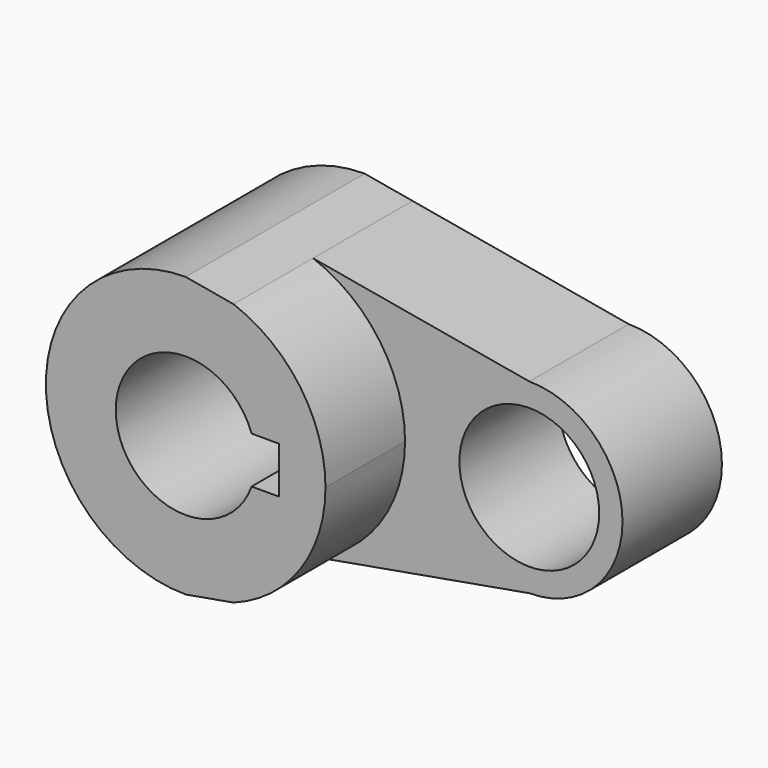
from build123d import *

# Parameters (mm, degrees)
F0_R     = 14.2875
F1_DEPTH = 25.4
F2_DEPTH = 45.72


with BuildPart() as f1:
    # F0 (on Front) → F1 (new body)
    with BuildSketch(Plane.XZ):
        with BuildLine():
            Line((9.780704698, 26.8489932886), (0, 28.575))
            ThreePointArc((0, 28.575), (-28.575, 0), (0, -28.575))
            Line((0, -28.575), (9.780704698, -26.8489932886))
            ThreePointArc((9.780704698, -26.8489932886), (23.4095521288, -16.3866864902), (28.575, 0))
            ThreePointArc((28.575, 0), (23.4095521288, 16.3866864902), (9.780704698, 26.8489932886))
        make_face()
        with BuildLine():
            ThreePointArc((-13.4703841816, 4.7625), (0, 14.2875), (13.4703841816, 4.7625))
            Line((13.4703841816, 4.7625), (19.05, 4.7625))
            Line((19.05, 4.7625), (19.05, -4.7625))
            Line((19.05, -4.7625), (13.4703841816, -4.7625))
            ThreePointArc((13.4703841816, -4.7625), (0, -14.2875), (-13.4703841816, -4.7625))
            Line((-13.4703841816, -4.7625), (-19.05, -4.7625))
            Line((-19.05, -4.7625), (-19.05, 4.7625))
            Line((-19.05, 4.7625), (-13.4703841816, 4.7625))
        make_face(mode=Mode.SUBTRACT)
        with BuildLine():
            Line((53.975, 19.05), (9.780704698, 26.8489932886))
            ThreePointArc((9.780704698, 26.8489932886), (23.4095521288, 16.3866864902), (28.575, 0))
            ThreePointArc((28.575, 0), (23.4095521288, -16.3866864902), (9.780704698, -26.8489932886))
            Line((9.780704698, -26.8489932886), (53.975, -19.05))
            ThreePointArc((53.975, -19.05), (34.925, 0), (53.975, 19.05))
        make_face()
        with BuildLine():
            ThreePointArc((73.025, 0), (67.4453841816, 13.4703841816), (53.975, 19.05))
            ThreePointArc((53.975, 19.05), (34.925, 0), (53.975, -19.05))
            ThreePointArc((53.975, -19.05), (67.4453841816, -13.4703841816), (73.025, 0))
        make_face()
        with Locations((53.975, 0)):
            Circle(F0_R, mode=Mode.SUBTRACT)
        with BuildLine():
            ThreePointArc((-13.4703841816, -4.7625), (-14.2875, 0), (-13.4703841816, 4.7625))
            Line((-13.4703841816, 4.7625), (-19.05, 4.7625))
            Line((-19.05, 4.7625), (-19.05, -4.7625))
            Line((-19.05, -4.7625), (-13.4703841816, -4.7625))
        make_face()
    extrude(amount=F1_DEPTH)

    # F0 (on Front) → F2 (join)
    with BuildSketch(Plane.XZ):
        with BuildLine():
            Line((9.780704698, 26.8489932886), (0, 28.575))
            ThreePointArc((0, 28.575), (-28.575, 0), (0, -28.575))
            Line((0, -28.575), (9.780704698, -26.8489932886))
            ThreePointArc((9.780704698, -26.8489932886), (23.4095521288, -16.3866864902), (28.575, 0))
            ThreePointArc((28.575, 0), (23.4095521288, 16.3866864902), (9.780704698, 26.8489932886))
        make_face()
        with BuildLine():
            ThreePointArc((-13.4703841816, 4.7625), (0, 14.2875), (13.4703841816, 4.7625))
            Line((13.4703841816, 4.7625), (19.05, 4.7625))
            Line((19.05, 4.7625), (19.05, -4.7625))
            Line((19.05, -4.7625), (13.4703841816, -4.7625))
            ThreePointArc((13.4703841816, -4.7625), (0, -14.2875), (-13.4703841816, -4.7625))
            Line((-13.4703841816, -4.7625), (-19.05, -4.7625))
            Line((-19.05, -4.7625), (-19.05, 4.7625))
            Line((-19.05, 4.7625), (-13.4703841816, 4.7625))
        make_face(mode=Mode.SUBTRACT)
        with BuildLine():
            ThreePointArc((-13.4703841816, -4.7625), (-14.2875, 0), (-13.4703841816, 4.7625))
            Line((-13.4703841816, 4.7625), (-19.05, 4.7625))
            Line((-19.05, 4.7625), (-19.05, -4.7625))
            Line((-19.05, -4.7625), (-13.4703841816, -4.7625))
        make_face()
    extrude(amount=F2_DEPTH)


solid = f1.part
